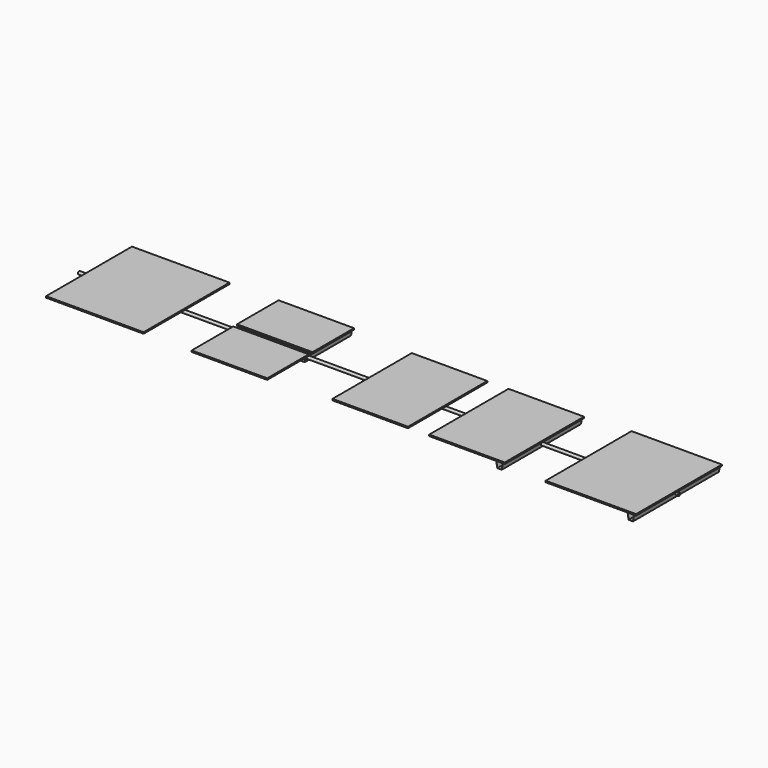
from build123d import *

# Parameters (mm, degrees)
F0_W      = 826.5
F0_H      = 910.1
F1_DEPTH  = 12
F0_W_2    = 640
F0_H_2    = 840
F2_DEPTH  = 12
F3_DEPTH  = 12
F0_W_3    = 766
F4_DEPTH  = 12
F5_W      = 910.1
F5_H      = 51
F5_R      = 12.5
F6_DEPTH  = 10
F7_W      = 840
F7_H      = 51
F7_R      = 12.5
F8_DEPTH  = 10
F0_H_3    = 440
F9_DEPTH  = 12
F10_DEPTH = 12
F11_W     = 440
F11_H     = 51
F11_W_2   = 50
F11_R     = 12.5
F12_DEPTH = 10
F14_DEPTH = 490
F15_R     = 12.5
F16_REACH = 1950.671915624
F18_DEPTH = 840
F19_R     = 12.5
F20_REACH = 3931.916736964
F22_DEPTH = 910.1
F23_R     = 12.5
F24_REACH = 5072.9586354833
F27_R     = 12.5
F28_DEPTH = 5000.8404067762


# Not quite as in the source:
# - a pattern or mirror of a feature is missing from the dataset's text; its kind, count and spacing are read off the source's solid


with BuildPart() as f1:
    # F0 (on Top) → F1 (new body)
    with BuildSketch(Plane.XY):
        with Locations((-2278.6802578143, 0)):
            Rectangle(F0_W, F0_H)
    extrude(amount=F1_DEPTH)


with BuildPart() as f2:
    # F0 (on Top) → F2 (new body)
    with BuildSketch(Plane.XY):
        with Locations((27.8577636927, 0)):
            Rectangle(F0_W_2, F0_H_2)
    extrude(amount=F2_DEPTH)


with BuildPart() as f3:
    # F0 (on Top) → F3 (new body)
    with BuildSketch(Plane.XY):
        with Locations((847.8672504425, 0)):
            Rectangle(F0_W_2, F0_H_2)
    extrude(amount=F3_DEPTH)


with BuildPart() as f4:
    # F0 (on Top) → F4 (new body)
    with BuildSketch(Plane.XY):
        with Locations((1925.9091489618, 0)):
            Rectangle(F0_W_3, F0_H)
    extrude(amount=F4_DEPTH)


with BuildPart() as f6:
    # F5 (on face) → F6 (new body)
    with BuildSketch(Plane.YZ.offset(2308.9091489618)):
        with Locations((0, -25.5)):
            Rectangle(F5_W, F5_H)
        with Locations((0, -25.5)):
            Circle(F5_R, mode=Mode.SUBTRACT)
    extrude(amount=-F6_DEPTH)


with BuildPart() as f8:
    # F7 (on face) → F8 (new body)
    with BuildSketch(Plane.YZ.offset(1167.8672504425)):
        with Locations((0, -25.5)):
            Rectangle(F7_W, F7_H)
        with Locations((0, -25.5)):
            Circle(F7_R, mode=Mode.SUBTRACT)
    extrude(amount=-F8_DEPTH)


with BuildPart() as f9:
    # F0 (on Top) → F9 (new body)
    with BuildSketch(Plane.XY):
        with Locations((-1133.3775708974, 240)):
            Rectangle(F0_W_2, F0_H_3)
    extrude(amount=F9_DEPTH)


with BuildPart() as f10:
    # F0 (on Top) → F10 (new body)
    with BuildSketch(Plane.XY):
        with Locations((-1133.3775708974, -240)):
            Rectangle(F0_W_2, F0_H_3)
    extrude(amount=F10_DEPTH)


with BuildPart() as f12:
    # F11 (on face) → F12 (new body)
    with BuildSketch(Plane.YZ.offset(-813.3775708974)):
        with Locations((240, -25.5)):
            Rectangle(F11_W, F11_H)
        with Locations((-5, -25.5)):
            Rectangle(F11_W_2, F11_H)
        with Locations((-5, -25.5)):
            Circle(F11_R, mode=Mode.SUBTRACT)
    extrude(amount=-F12_DEPTH)


with BuildPart() as f14:
    # F13 (on face) → F14 (new body, through all)
    with BuildSketch(Plane.XZ.offset(30)):
        Polygon((-800.4310302851, -50), (-836.3241115098, -50), (-845.1404605452, 0), (-860.1404605452, 0), (-860.1404605452, -1), (-845.9795601764, -1), (-837.163211141, -51), (-799.5919306539, -51), (-790.7755816185, -1), (-776.6146812496, -1), (-776.6146812496, 0), (-791.6146812496, 0), align=None)
    extrude(amount=-F14_DEPTH)

    f16_end = f14.faces().sort_by_distance((-841.5713856587, 215, -26))[0]
    # F15 (on face) → F16 (cut, up to a face of the model that its end follows)
    with BuildSketch(Plane.YZ.offset(-776.6146812496)):
        with Locations((-5, -25.5)):
            Circle(F15_R)
    f16_long = extrude(amount=-F16_REACH, mode=Mode.PRIVATE)
    add(split(f16_long, bisect_by=f16_end, keep=Keep.BOTTOM, mode=Mode.PRIVATE), mode=Mode.SUBTRACT)


with BuildPart() as f18:
    # F17 (on face) → F18 (new body, through all)
    with BuildSketch(Plane.XZ.offset(420)):
        Polygon((1180.8137910549, -50), (1144.9207098301, -50), (1136.1043607947, 0), (1121.1043607947, 0), (1121.1043607947, -1), (1135.2652611635, -1), (1144.081610199, -51), (1181.6528906861, -51), (1190.4692397215, -1), (1204.6301400903, -1), (1204.6301400903, 0), (1189.6301400903, 0), align=None)
    extrude(amount=-F18_DEPTH)

    f20_end = f18.faces().sort_by_distance((1139.6734356812, 0, -26))[0]
    # F19 (on face) → F20 (cut, up to a face of the model that its end follows)
    with BuildSketch(Plane.YZ.offset(1204.6301400903)):
        with Locations((0, -25.5)):
            Circle(F19_R)
    f20_long = extrude(amount=-F20_REACH, mode=Mode.PRIVATE)
    add(split(f20_long, bisect_by=f20_end, keep=Keep.BOTTOM, mode=Mode.PRIVATE), mode=Mode.SUBTRACT)


with BuildPart() as f22:
    # F21 (on face) → F22 (new body, through all)
    with BuildSketch(Plane.XZ.offset(455.05)):
        Polygon((2321.8556895742, -50), (2285.9626083495, -50), (2277.146259314, 0), (2262.146259314, 0), (2262.146259314, -1), (2276.3071596829, -1), (2285.1235087183, -51), (2322.6947892054, -51), (2331.5111382408, -1), (2345.6720386096, -1), (2345.6720386096, 0), (2330.6720386096, 0), align=None)
    extrude(amount=-F22_DEPTH)

    f24_end = f22.faces().sort_by_distance((2280.7153342006, 0, -26))[0]
    # F23 (on face) → F24 (cut, up to a face of the model that its end follows)
    with BuildSketch(Plane.YZ.offset(2345.6720386096)):
        with Locations((0, -25.5)):
            Circle(F23_R)
    f24_long = extrude(amount=-F24_REACH, mode=Mode.PRIVATE)
    add(split(f24_long, bisect_by=f24_end, keep=Keep.BOTTOM, mode=Mode.PRIVATE), mode=Mode.SUBTRACT)


with BuildPart() as f14_1:
    # F25: moved
    add(f14.part.moved(Location((-39, 0, 0))))


with BuildPart() as f18_1:
    # F25: moved
    add(f18.part.moved(Location((-39, 0, 0))))


with BuildPart() as f22_1:
    # F25: moved
    add(f22.part.moved(Location((-39, 0, 0))))


with BuildPart() as f28:
    # F27 (on face) → F28 (new body, through all)
    with BuildSketch(Plane.YZ.offset(2308.9091489618)):
        with Locations((0, -25.5)):
            Circle(F27_R)
    extrude(amount=-F28_DEPTH)

    # F28_copies: F28 across plane


with BuildPart() as f28_1:
    add(f28.part)
    add(f28.part.mirror(Plane(origin=(-233.671502, 0, 0), x_dir=(0, 0, -1), z_dir=(-1, 0, 0))))


solid = Compound([f1.part, f2.part, f3.part, f4.part, f9.part, f10.part, f14_1.part, f18_1.part, f22_1.part, f28_1.part])
